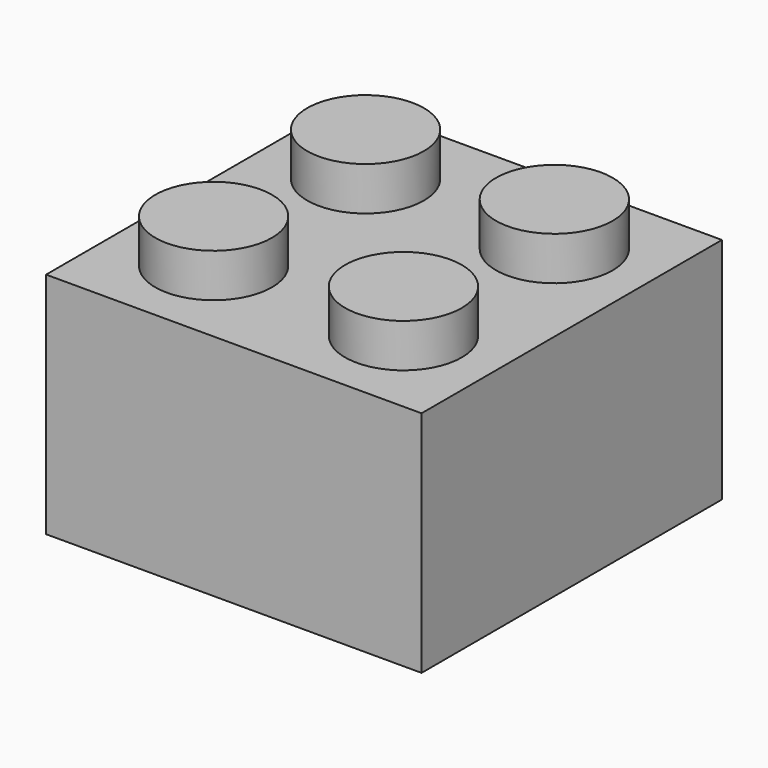
from build123d import *

# Parameters (mm, degrees)
F0_W     = 15.7734
F0_H     = 15.7734
F1_DEPTH = 9.6012
F2_R     = 2.4511
F3_DEPTH = 11.43
F4_W     = 13.2842
F4_H     = 13.2842
F4_R     = 3.2258
F5_DEPTH = 7.62
F6_R     = 2.4511
F7_DEPTH = 7.62


# Not quite as in the source:
# - a feature names something its author has since deleted; it is built from what else it names


with BuildPart() as f1:
    # F0 (on Top) → F1 (new body)
    with BuildSketch(Plane.XY):
        Rectangle(F0_W, F0_H)
    extrude(amount=F1_DEPTH)

    # F2 (on face) → F3 (join)
    with BuildSketch(Plane.XY):
        with Locations((-3.94462, 3.9624)):
            Circle(F2_R)
        with Locations((3.9878, 3.9624)):
            Circle(F2_R)
        with Locations((-3.9878, -3.9624)):
            Circle(F2_R)
        with Locations((3.9878, -3.9624)):
            Circle(F2_R)
    extrude(amount=F3_DEPTH)

    # F4 (on face) → F5 (cut)
    with BuildSketch(Plane(origin=(0, 0, 0), x_dir=(1, 0, 0), z_dir=(0, 0, -1))):
        Rectangle(F4_W, F4_H)
        Circle(F4_R, mode=Mode.SUBTRACT)
    extrude(amount=-F5_DEPTH, mode=Mode.SUBTRACT)

    # F6 (on face) → F7 (cut)
    with BuildSketch(Plane(origin=(0, 0, 0), x_dir=(1, 0, 0), z_dir=(0, 0, -1))):
        Circle(F6_R)
    extrude(amount=-F7_DEPTH, mode=Mode.SUBTRACT)


solid = f1.part
